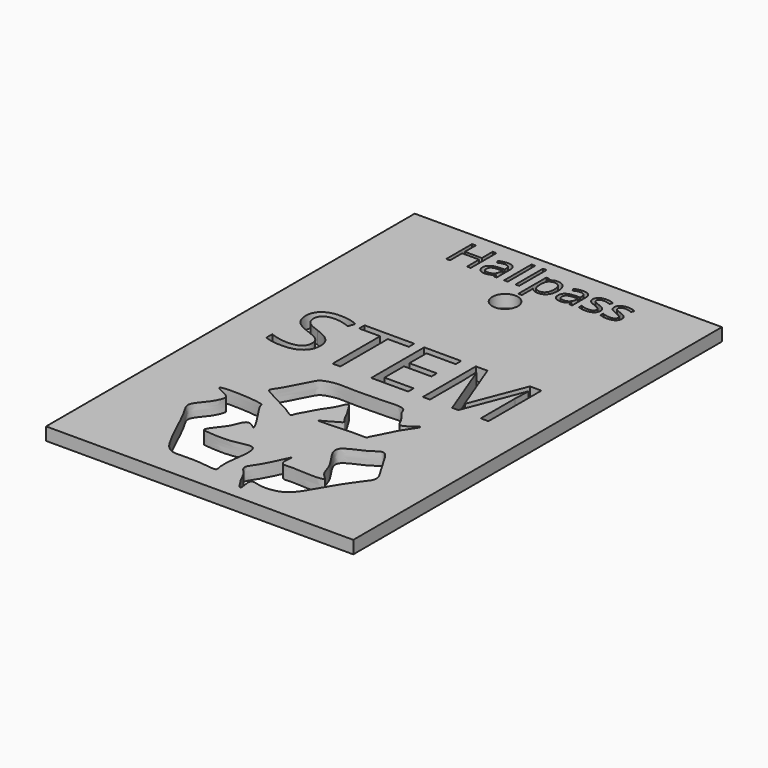
from build123d import *

# Parameters (mm, degrees)
F0_W          = 76.2
F0_H          = 114.3
F1_DEPTH      = 3.175
F2_R          = 3.175
F3_DEPTH      = 3.175
F4_TEXT_SIZE  = 23.0140518397
F5_DEPTH      = 3.175
F7_DEPTH      = 3.175
F9_DEPTH      = 3.175
F11_DEPTH     = 3.175
F12_TEXT_SIZE = 11.1896699915
F13_DEPTH     = 3.175


# Not quite as in the source:
# - Text() gives the source's letters only with a copy of the font that has no kerning and outlines rounded to 1/6400 em; it was checked with that copy


with BuildPart() as f1:
    # F0 (on Top) → F1 (new body)
    with BuildSketch(Plane.XY):
        with Locations((1.1512245983, 1.9336916171)):
            Rectangle(F0_W, F0_H)
    extrude(amount=F1_DEPTH)

    # F2 (on face) → F3 (cut)
    with BuildSketch(Plane.XY.offset(3.175)):
        with Locations((-0.2534315848, 41.2279086976)):
            Circle(F2_R)
    extrude(amount=-F3_DEPTH, mode=Mode.SUBTRACT)

    # F4 (on face) → F5 (cut)
    with BuildSketch(Plane.XY.offset(3.175)):
        with Locations((-28.0902925879, 0)):
            Text('STEM', F4_TEXT_SIZE, font='Open Sans', text_align=(TextAlign.LEFT, TextAlign.BOTTOM))
    extrude(amount=-F5_DEPTH, mode=Mode.SUBTRACT)

    # F6 (on Top) → F7 (cut)
    with BuildSketch(Plane.XY):
        with BuildLine():
            add(Edge.make_bspline(
                [(-12.7017358318, -16.3541063666), (-12.5153254399, -16.8008009028), (-10.5565220334, -17.5956869314), (-8.9783806135, -18.6192156072), (-7.0419219355, -19.5744765175), (-4.9414926935, -20.6702388871), (-2.755812813, -22.2889694606), (-2.6616770475, -21.1767757069), (-1.7627117206, -19.7233672259), (-1.045067592, -18.468442228), (-0.0545453472, -16.2529523175), (1.8376026727, -14.1193898376), (2.8321001747, -10.8563611614), (3.670946653, -12.0062406852), (4.3489959401, -13.3571125888), (5.3387311883, -14.6316368424), (6.0378056936, -16.6436168129), (7.4674950548, -17.8063449272), (5.708537856, -18.5525708435), (3.9274515655, -19.8071070113), (2.0658969333, -20.4778504298), (4.5756471943, -20.4151436126), (6.5111812736, -20.3792641236), (8.6884821307, -20.1785956205), (10.8898244122, -20.1323929785), (13.233567028, -20.0896056276), (14.5982764148, -20.2258495299), (14.5516176841, -19.5534468366), (15.2140079552, -18.6543070652), (15.7448384621, -17.2538253417), (16.7981632396, -15.5484797814), (17.5886664271, -13.5896912965), (19.1062674987, -11.6568068585), (20.2153006123, -9.7429367299), (18.8368875061, -10.5763813341), (16.0874877398, -12.8256978018), (15.3943124812, -10.5295927124), (14.3866031932, -9.1678932616), (13.1011668413, -7.8069838892), (12.8912083452, -6.264621148), (10.9456223015, -5.7472863262), (8.663041097, -6.0352747608), (4.6633804284, -5.9883416771), (0.0190827994, -6.2281658534), (-3.8252722442, -5.7925167611), (-6.9833928548, -6.6296746761), (-8.0781972782, -7.4854151169), (-9.0211629117, -9.5735062533), (-10.4221608239, -12.167302008), (-12.0169011942, -15.0921347187), (-12.839649753, -16.0236237448), (-12.7017358318, -16.3541063666)],
                knots=[0, 0, 0, 0, 0.0221889049, 0.04321626, 0.0640685623, 0.0878709965, 0.1092175606, 0.1209657605, 0.14009215, 0.15791759, 0.1800220673, 0.2061440473, 0.2297904478, 0.2425980716, 0.2610041243, 0.2796259243, 0.3012897093, 0.3179687001, 0.3349108376, 0.3584301484, 0.3735244472, 0.3919590706, 0.4138363225, 0.43501569, 0.4568929329, 0.4797983649, 0.4950292762, 0.5049082866, 0.5200025883, 0.5380142733, 0.558537141, 0.5797165122, 0.6037538207, 0.6213761231, 0.6357646718, 0.6612406422, 0.6797508217, 0.6994856689, 0.7191269038, 0.7361540765, 0.7551602306, 0.777387174, 0.8065222511, 0.8382470058, 0.8673250877, 0.8928441578, 0.9094195454, 0.9307661096, 0.9565079238, 0.9835837538, 1, 1, 1, 1], degree=3))
        make_face()
    extrude(amount=F7_DEPTH, mode=Mode.SUBTRACT)

    # F8 (on face) → F9 (cut)
    with BuildSketch(Plane.XY.offset(3.175)):
        with BuildLine():
            add(Edge.make_bspline(
                [(13.2336784154, -27.1470695734), (13.945215269, -25.9930010546), (18.4013506627, -24.7356525195), (21.0361769604, -21.7763591782), (23.4562093961, -26.2124327205), (25.1738760211, -29.1460294217), (27.3831196653, -32.4168897929), (25.1098708534, -35.1106833758), (21.1692583025, -40.8691855635), (18.2303744482, -46.8320395779), (14.9361828119, -48.7957924297), (10.8143603868, -48.9568568131), (7.568770489, -47.5740658547), (9.367850004, -53.5708319552), (6.2444931491, -49.0017909645), (5.5111609289, -46.6705375915), (3.1937192462, -44.8004195747), (4.717022108, -42.7700847206), (6.4940306157, -39.8367718102), (9.0125802326, -33.7223052474), (7.7077863077, -39.2732111622), (10.6694069711, -38.8403738877), (14.090173818, -39.1272067285), (17.652393649, -39.2263386582), (19.4456811567, -38.812195572), (17.675691425, -37.5694906726), (16.8550253137, -35.8214255608), (16.220570782, -33.4207815241), (13.7135229878, -30.2776022985), (12.721326152, -27.9780730763), (13.2336784154, -27.1470695734)],
                knots=[0, 0, 0, 0, 0.0473772607, 0.0819684062, 0.1207247129, 0.1599681067, 0.1959609092, 0.2300677504, 0.283272854, 0.3342699551, 0.3715361986, 0.4123907892, 0.4412731, 0.4763120571, 0.5107773428, 0.5458442598, 0.5760560608, 0.6033948509, 0.6445290408, 0.6837225365, 0.7165788428, 0.7450267156, 0.7834052785, 0.8217731786, 0.842248854, 0.8665568731, 0.8946856561, 0.9254703447, 0.9658853275, 1, 1, 1, 1], degree=3))
        make_face()
    extrude(amount=-F9_DEPTH, mode=Mode.SUBTRACT)

    # F10 (on face) → F11 (cut)
    with BuildSketch(Plane.XY.offset(3.175)):
        with BuildLine():
            add(Edge.make_bspline(
                [(-20.8570044488, -21.4911028743), (-20.3741367352, -20.7791745425), (-9.63203931, -21.3265461263), (-10.1720528547, -22.676369769), (-7.5254005735, -26.2579250404), (-4.099961219, -31.9496997764), (-7.6427750532, -28.2784574818), (-8.9503750548, -31.9776523167), (-9.7025692122, -33.4858909779), (-13.034898614, -37.3372098296), (-10.6577820307, -37.5532870902), (-4.7898882355, -38.0940776345), (1.4600247369, -35.5332746363), (-0.2266349465, -44.1569673903), (-0.1708720514, -47.5111184175), (0.5235639099, -49.3507079756), (-5.7089376199, -47.8082298299), (-11.5974888703, -49.0345569382), (-14.2882437184, -45.3525106635), (-16.5761496486, -40.6003638596), (-19.7920299372, -33.5745050429), (-21.923041809, -30.6993697778), (-18.584007954, -27.4058575853), (-17.2583938783, -24.5508842631), (-17.3600754941, -23.1692305901), (-21.1366085546, -21.9033443206), (-20.8570044488, -21.4911028743)],
                knots=[0, 0, 0, 0, 0.0692375841, 0.0887227432, 0.1358539158, 0.1803415064, 0.21216543, 0.2474160685, 0.2803425026, 0.3230672492, 0.3468804411, 0.4011801223, 0.4470415099, 0.5023023257, 0.5439854443, 0.5645088132, 0.6137195004, 0.6665635058, 0.7079467544, 0.7583759435, 0.8182015768, 0.8549377945, 0.8985079536, 0.936094852, 0.9599080405, 1, 1, 1, 1], degree=3))
        make_face()
    extrude(amount=-F11_DEPTH, mode=Mode.SUBTRACT)

    # F12 (on face) → F13 (cut)
    with BuildSketch(Plane.XY.offset(3.175)):
        with Locations((-21.3915593922, 48.0586700141)):
            Text('Hallpass', F12_TEXT_SIZE, font='Open Sans', text_align=(TextAlign.LEFT, TextAlign.BOTTOM))
    extrude(amount=-F13_DEPTH, mode=Mode.SUBTRACT)


solid = f1.part
